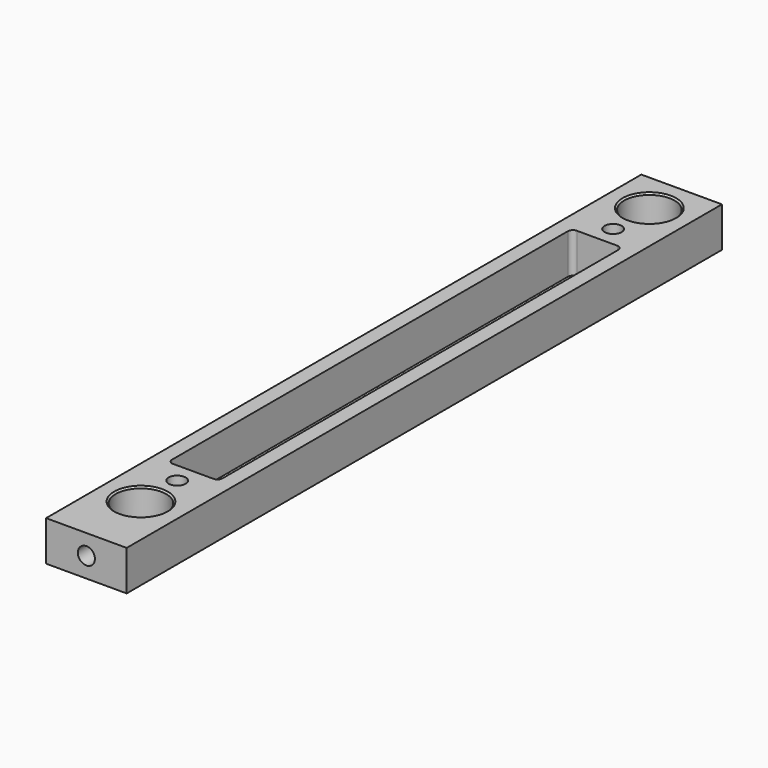
from build123d import *

# Parameters (mm, degrees)
F0_W     = 12.7625
F0_H     = 117.8206766
F0_R     = 4
F0_R_2   = 1.35255
F0_W_2   = 8
F0_H_2   = 79.9424962
F1_DEPTH = 6.35
F2_R     = 0.79375
F3_SIZE  = 0.254
F4_R     = 1.35255
F5_DEPTH = 8.0325436313


# Not quite as in the source:
# - a feature names something its author has since deleted; it is built from what else it names


with BuildPart() as f1:
    # F0 (on Top) → F1 (new body)
    with BuildSketch(Plane.XY):
        with Locations((0, -2.2078402)):
            Rectangle(F0_W, F0_H)
        with Locations((0, -50.3212481)):
            Circle(F0_R, mode=Mode.SUBTRACT)
        with Locations((0, -43.1462481)):
            Circle(F0_R_2, mode=Mode.SUBTRACT)
        Rectangle(F0_W_2, F0_H_2, mode=Mode.SUBTRACT)
        with Locations((0, 43.1462481)):
            Circle(F0_R_2, mode=Mode.SUBTRACT)
        with Locations((0, 50.3212481)):
            Circle(F0_R, mode=Mode.SUBTRACT)
    extrude(amount=F1_DEPTH)

    # F2
    f2_edges = [f1.edges().sort_by_distance(p)[0] for p in [
        (4, -39.971248, 3.175),
        (-4, -39.971248, 3.175),
        (-4, 39.971248, 3.175),
        (4, 39.971248, 3.175),
    ]]
    fillet(f2_edges, radius=F2_R)

    # F3
    f3_edges = [f1.edges().sort_by_distance(p)[0] for p in [
        (-4, 50.321248, 6.35),
        (-4, -50.321248, 6.35),
    ]]
    chamfer(f3_edges, length=F3_SIZE)

    # F4 (on face) → F5 (cut, up to face)
    with BuildSketch(Plane.XZ.offset(61.1181785)):
        with Locations((0, 3.175)):
            Circle(F4_R)
    extrude(amount=-F5_DEPTH, mode=Mode.SUBTRACT)


solid = f1.part
